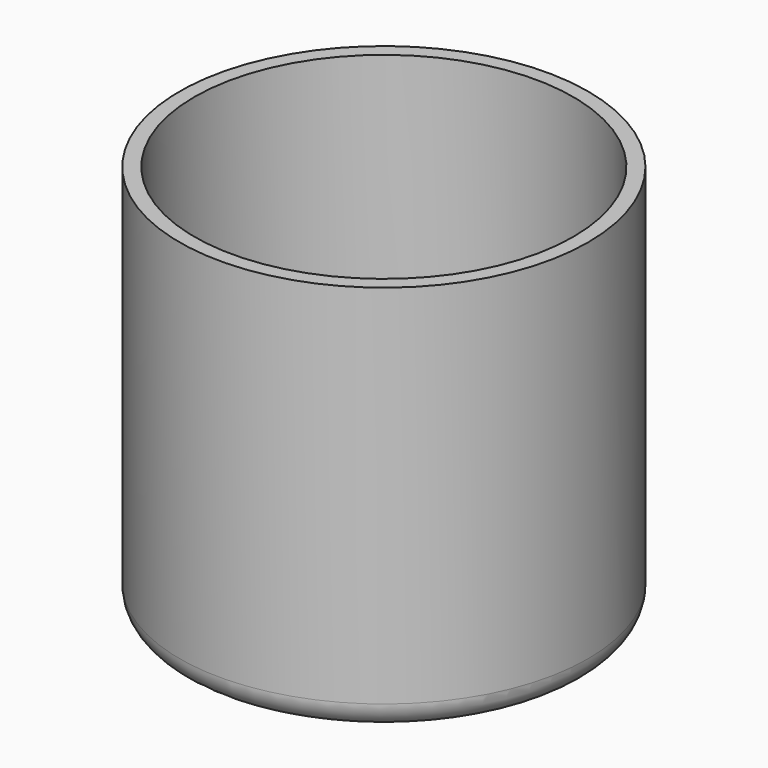
from build123d import *

# Parameters (mm, degrees)
F0_R     = 55
F0_R_2   = 51
F0_R_3   = 47
F1_DEPTH = 5
F2_DEPTH = 50
F3_DEPTH = 100
F4_R     = 10
F5_DEPTH = 25
F6_DEPTH = 25
F7_DEPTH = 25


# Not quite as in the source:
# - a fillet or chamfer that OpenCascade refuses, or shapes differently, is made with other operations: its cross-section is extruded or revolved along the edge and cut away or added


with BuildPart() as f1:
    # F0 (on Top) → F1 (new body)
    with BuildSketch(Plane.XY):
        Circle(F0_R)
        Circle(F0_R_2, mode=Mode.SUBTRACT)
        Circle(F0_R_2)
        Circle(F0_R_3, mode=Mode.SUBTRACT)
        Circle(F0_R_3)
    extrude(amount=F1_DEPTH)

    # F0 (on Top) → F2 (join)
    with BuildSketch(Plane.XY):
        Circle(F0_R_2)
        Circle(F0_R_3, mode=Mode.SUBTRACT)
    extrude(amount=F2_DEPTH)

    # F3 (add): a face of the model
    f3_faces = [f1.faces().sort_by_distance(p)[0] for p in [
        (-53.4443650814, 0, 5),
    ]]
    extrude(f3_faces, amount=F3_DEPTH)

    # F4
    f4_edges = [f1.edges().sort_by_distance(p)[0] for p in [
        (-55, 0, 0),
    ]]
    fillet(f4_edges, radius=F4_R)

    # F0 (on Top) → F5 (join)
    with BuildSketch(Plane.XY):
        Circle(F0_R)
        Circle(F0_R_2, mode=Mode.SUBTRACT)
    extrude(amount=F5_DEPTH)

    # F0 (on Top) → F6 (join)
    with BuildSketch(Plane.XY):
        Circle(F0_R)
        Circle(F0_R_2, mode=Mode.SUBTRACT)
    extrude(amount=F6_DEPTH)

    # F0 (on Top) → F7 (join)
    with BuildSketch(Plane.XY):
        Circle(F0_R)
        Circle(F0_R_2, mode=Mode.SUBTRACT)
    extrude(amount=F7_DEPTH)

    # F8: fillet of radius 7 on 1 edges, made by hand

    # F8_s1 → F8_t2 (revolve, cut)
    with BuildSketch(Plane.XZ):
        with BuildLine():
            ThreePointArc((55, 6.3245553203), (53.9160797831, 2.5828979336), (51, 0))
            Line((51, 0), (55, 0))
            Line((55, 0), (55, 6.3245553203))
        make_face()
    revolve(axis=Axis((0, 0, 0), (0, 0, 1)), mode=Mode.SUBTRACT)


solid = f1.part
